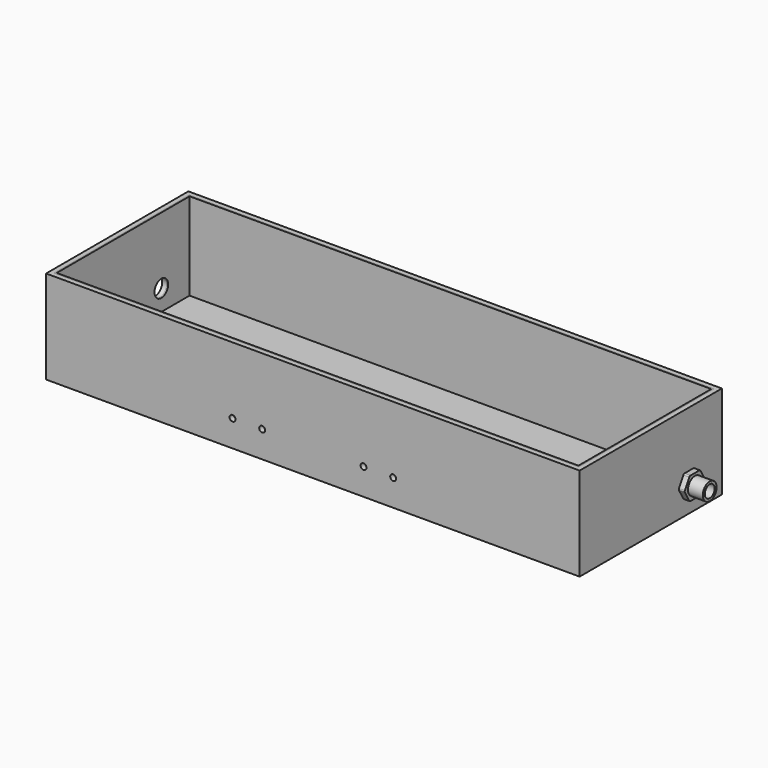
from build123d import *

# Parameters (mm, degrees)
F0_W      = 900
F0_H      = 300
F1_DEPTH  = 7.5
F2_W      = 900
F2_H      = 300
F2_W_2    = 885
F2_H_2    = 285
F3_DEPTH  = 150
F4_DEPTH  = 2.5
F5_W      = 885
F5_H      = 285
F5_W_2    = 880
F5_H_2    = 280
F6_DEPTH  = 147.5
F7_R      = 5
F8_DEPTH  = 25
F9_R      = 14.39
F10_DEPTH = 500
F11_R     = 14.39
F12_DEPTH = 25
F13_R     = 14.39
F13_R_2   = 10.39
F14_DEPTH = 10
F15_R     = 10.39
F16_DEPTH = 10
F17_R     = 14.6154428136
F17_R_2   = 10.39
F18_DEPTH = 25
F19_R     = 11.2359155228
F19_R_2   = 8.5030368104
F20_DEPTH = 50
F21_R     = 11.2359155228
F22_DEPTH = 10
F23_DEPTH = 50


with BuildPart() as f1:
    # F0 (on Top) → F1 (new body)
    with BuildSketch(Plane.XY):
        Rectangle(F0_W, F0_H)
    extrude(amount=F1_DEPTH)

    # F2 (on face) → F3 (join)
    with BuildSketch(Plane.XY.offset(7.5)):
        Rectangle(F2_W, F2_H)
        Rectangle(F2_W_2, F2_H_2, mode=Mode.SUBTRACT)
    extrude(amount=F3_DEPTH)


with BuildPart() as f4:
    # F4 (new): a face of the model
    f4_faces = [f1.part.faces().sort_by_distance(p)[0] for p in [
        (0, 0, 7.5),
    ]]
    extrude(f4_faces, amount=F4_DEPTH)

    # F5 (on face) → F6 (join)
    with BuildSketch(Plane.XY.offset(10)):
        Rectangle(F5_W, F5_H)
        Rectangle(F5_W_2, F5_H_2, mode=Mode.SUBTRACT)
    extrude(amount=F6_DEPTH)


with BuildPart() as f8_tool:
    # F7 (on face) → F8 (new body)
    with BuildSketch(Plane.XZ.offset(150)):
        with Locations((85.5, 44.781)):
            Circle(F7_R)
        with Locations((135.5, 44.781)):
            Circle(F7_R)
        with Locations((-85.5, 44.78)):
            Circle(F7_R)
        with Locations((-135.5, 44.78)):
            Circle(F7_R)
    extrude(amount=-F8_DEPTH)


with BuildPart() as f1_1:
    add(f1.part)

    # F8: cut by f8_tool
    add(f8_tool.part, mode=Mode.SUBTRACT)


with BuildPart() as f4_1:
    add(f4.part)

    # F8: cut by f8_tool
    add(f8_tool.part, mode=Mode.SUBTRACT)


with BuildPart() as f10_tool:
    # F9 (on face) → F10 (new body)
    with BuildSketch(Plane(origin=(-450, 0, 0), x_dir=(0, -1, 0), z_dir=(-1, 0, 0))):
        with Locations((-80.5, 45)):
            Circle(F9_R)
    extrude(amount=-F10_DEPTH)


with BuildPart() as f1_2:
    add(f1_1.part)

    # F10: cut by f10_tool
    add(f10_tool.part, mode=Mode.SUBTRACT)


with BuildPart() as f4_2:
    add(f4_1.part)

    # F10: cut by f10_tool
    add(f10_tool.part, mode=Mode.SUBTRACT)


with BuildPart() as f12_tool:
    # F11 (on face) → F12 (new body)
    with BuildSketch(Plane.YZ.offset(450)):
        with Locations((80.5, 44.5)):
            Circle(F11_R)
    extrude(amount=-F12_DEPTH)


with BuildPart() as f1_3:
    add(f1_2.part)

    # F12: cut by f12_tool
    add(f12_tool.part, mode=Mode.SUBTRACT)


with BuildPart() as f4_3:
    add(f4_2.part)

    # F12: cut by f12_tool
    add(f12_tool.part, mode=Mode.SUBTRACT)


with BuildPart() as f14:
    # F13 (on face) → F14 (new body)
    with BuildSketch(Plane.YZ.offset(450)):
        with Locations((80.5, 44.5)):
            Circle(F13_R)
        with Locations((80.5, 44.5)):
            Circle(F13_R_2, mode=Mode.SUBTRACT)
    extrude(amount=-F14_DEPTH)

    # F15 (on face) → F16 (join)
    with BuildSketch(Plane.YZ.offset(450)):
        with BuildLine():
            Line((89.7447234463, 63.5123307109), (71.2552765537, 63.5123307109))
            ThreePointArc((71.2552765537, 63.5123307109), (69.7552765537, 63.1104069222), (68.6572003424, 62.0123307109))
            Line((68.6572003424, 62.0123307109), (59.4124768961, 46))
            ThreePointArc((59.4124768961, 46), (59.0105531074, 44.5), (59.4124768961, 43))
            Line((59.4124768961, 43), (68.6572003424, 26.9876692891))
            ThreePointArc((68.6572003424, 26.9876692891), (69.7552765537, 25.8895930778), (71.2552765537, 25.4876692891))
            Line((71.2552765537, 25.4876692891), (89.7447234463, 25.4876692891))
            ThreePointArc((89.7447234463, 25.4876692891), (91.2447234463, 25.8895930778), (92.3427996576, 26.9876692891))
            Line((92.3427996576, 26.9876692891), (101.5875231039, 43))
            ThreePointArc((101.5875231039, 43), (101.9894468926, 44.5), (101.5875231039, 46))
            Line((101.5875231039, 46), (92.3427996576, 62.0123307109))
            ThreePointArc((92.3427996576, 62.0123307109), (91.2447234463, 63.1104069222), (89.7447234463, 63.5123307109))
        make_face()
        with Locations((80.5, 44.5)):
            Circle(F15_R, mode=Mode.SUBTRACT)
    extrude(amount=F16_DEPTH)

    # F17 (on face) → F18 (join)
    with BuildSketch(Plane.YZ.offset(460)):
        with Locations((80.5, 44.5)):
            Circle(F17_R)
        with Locations((80.5, 44.5)):
            Circle(F17_R_2, mode=Mode.SUBTRACT)
    extrude(amount=F18_DEPTH)

    # F19 (on face) → F20 (join)
    with BuildSketch(Plane(origin=(440, 0, 0), x_dir=(0, -1, 0), z_dir=(-1, 0, 0))):
        with Locations((-80.5, 44.5)):
            Circle(F19_R)
        with Locations((-80.5, 44.5)):
            Circle(F19_R_2, mode=Mode.SUBTRACT)
    extrude(amount=F20_DEPTH)

    # F21 (on face) → F22 (join)
    with BuildSketch(Plane(origin=(440, 0, 0), x_dir=(0, -1, 0), z_dir=(-1, 0, 0))):
        with BuildLine():
            Line((-71.2552765537, 63.5123307109), (-89.7447234463, 63.5123307109))
            ThreePointArc((-89.7447234463, 63.5123307109), (-91.2447234463, 63.1104069222), (-92.3427996576, 62.0123307109))
            Line((-92.3427996576, 62.0123307109), (-101.5875231039, 46))
            ThreePointArc((-101.5875231039, 46), (-101.9894468926, 44.5), (-101.5875231039, 43))
            Line((-101.5875231039, 43), (-92.3427996576, 26.9876692891))
            ThreePointArc((-92.3427996576, 26.9876692891), (-91.2447234463, 25.8895930778), (-89.7447234463, 25.4876692891))
            Line((-89.7447234463, 25.4876692891), (-71.2552765537, 25.4876692891))
            ThreePointArc((-71.2552765537, 25.4876692891), (-69.7552765537, 25.8895930778), (-68.6572003424, 26.9876692891))
            Line((-68.6572003424, 26.9876692891), (-59.4124768961, 43))
            ThreePointArc((-59.4124768961, 43), (-59.0105531074, 44.5), (-59.4124768961, 46))
            Line((-59.4124768961, 46), (-68.6572003424, 62.0123307109))
            ThreePointArc((-68.6572003424, 62.0123307109), (-69.7552765537, 63.1104069222), (-71.2552765537, 63.5123307109))
        make_face()
        with Locations((-80.5, 44.5)):
            Circle(F21_R, mode=Mode.SUBTRACT)
    extrude(amount=F22_DEPTH)

    # F23 (add): a face of the model
    f23_faces = [f14.faces().sort_by_distance(p)[0] for p in [
        (390, 91.4181158404, 44.5),
    ]]
    extrude(f23_faces, amount=F23_DEPTH)


solid = Compound([f1_3.part, f4_3.part, f14.part])
